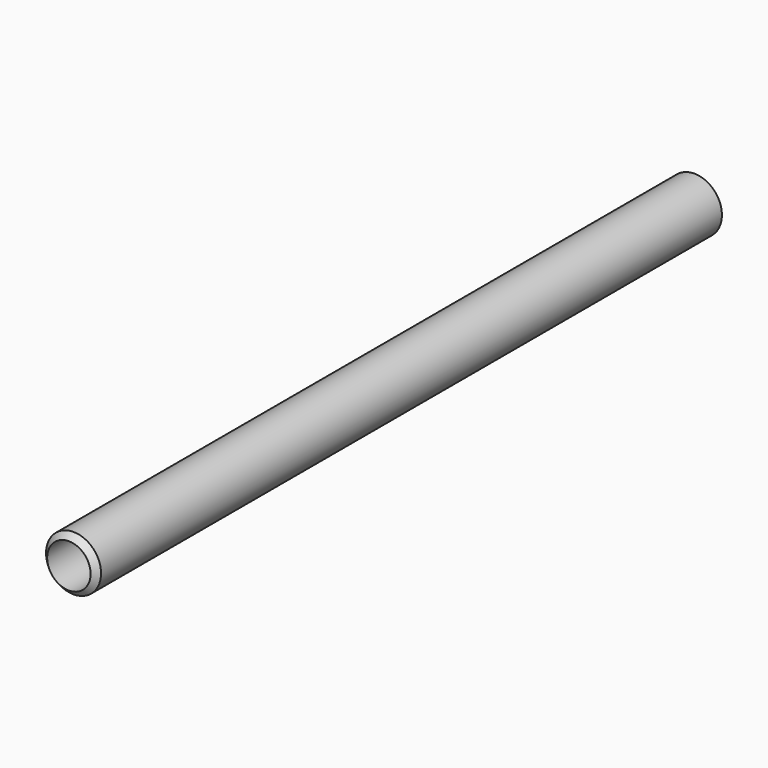
from build123d import *

# Parameters (mm, degrees)
F0_R          = 24.13
F0_R_2        = 19.05
F1_DEPTH      = 228.6
F1_DEPTH_BACK = 457.2
F2_SIZE       = 5.07999


# Not quite as in the source:
# - a fillet or chamfer is up to 0.001 mm smaller than in the source, because OpenCascade refuses the exact size


with BuildPart() as f1:
    # F0 (on Front) → F1 (new body, two sides)
    with BuildSketch(Plane.XZ) as f1_sk:
        Circle(F0_R)
        Circle(F0_R_2, mode=Mode.SUBTRACT)
    extrude(amount=F1_DEPTH)
    extrude(f1_sk.sketch, amount=-F1_DEPTH_BACK)

    # F2 (size 5.08 in the source; OpenCascade refuses exactly that, so slightly less here)
    f2_edges = [f1.edges().sort_by_distance(p)[0] for p in [
        (-24.13, -228.6, 0),
    ]]
    chamfer(f2_edges, length=F2_SIZE)


solid = f1.part
